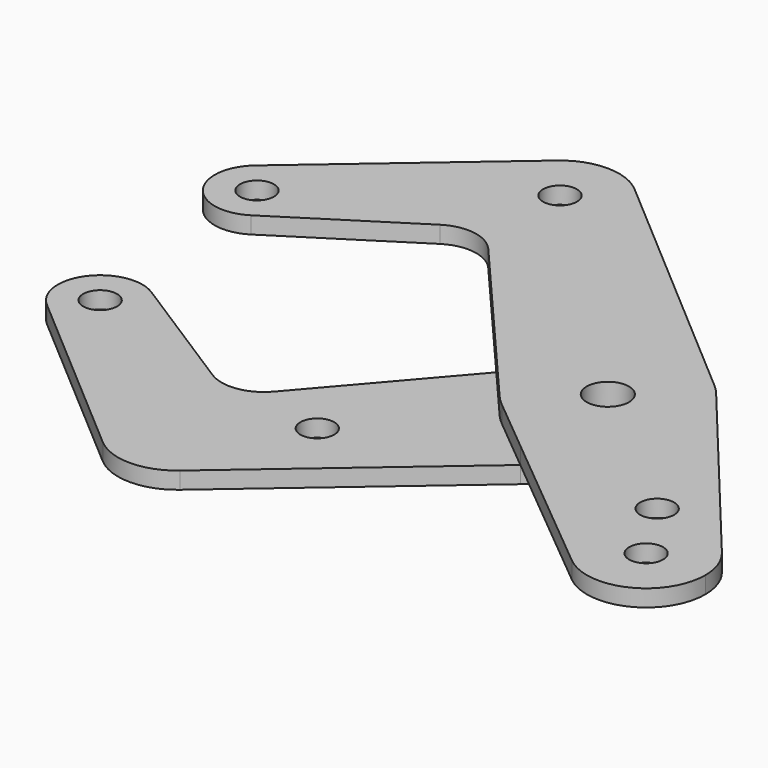
from build123d import *

# Parameters (mm, degrees)
F0_R     = 3.175
F0_R_2   = 3.9751
F1_DEPTH = 3.175
F2_DEPTH = 3.175


# Not quite as in the source:
# - after a boolean that leaves OpenCascade's solid faulty, fix() repairs it


with BuildPart() as f1:
    # F0 (on Top) → F1 (new body)
    with BuildSketch(Plane.XY):
        with BuildLine():
            Line((0.1954344954, -20.7710836138), (-10.1235074968, -12.2282550252))
            ThreePointArc((-10.1235074968, -12.2282550252), (-11.1192092809, -11.3304373246), (-12.0356034274, -10.3518054047))
            Line((-12.0356034274, -10.3518054047), (-20.9391765456, 0))
            Line((-20.9391765456, 0), (-42.5571087943, -25.134249466))
            ThreePointArc((-42.5571087943, -25.134249466), (-47.4235249822, -27.815033629), (-52.8569612369, -26.6546971654))
            Line((-52.8569612369, -26.6546971654), (-76.3196547531, -11.7034610596))
            ThreePointArc((-76.3196547531, -11.7034610596), (-73.6260110422, -14.5799404883), (-72.6477527528, -18.3973821792))
            ThreePointArc((-72.6477527528, -18.3973821792), (-77.2746501981, -25.611522251), (-85.7611554551, -24.4151838929))
            Line((-85.7611554551, -24.4151838929), (-52.1475443887, -53.3262030046))
            ThreePointArc((-52.1475443887, -53.3262030046), (-49.5361241819, -34.8014845049), (-33.7887806053, -44.9012806053))
            ThreePointArc((-33.7887806053, -44.9012806053), (-34.8014845049, -49.5361241819), (-37.655016822, -53.3262030046))
            Line((-37.655016822, -53.3262030046), (0.1954344954, -20.7710836138))
        make_face()
        with Locations((-30.2993841525, -30.2993841525)):
            Circle(F0_R, mode=Mode.SUBTRACT)
        with BuildLine():
            ThreePointArc((-52.1475443887, -53.3262030046), (-44.9012806053, -56.0137806053), (-37.655016822, -53.3262030046))
            ThreePointArc((-37.655016822, -53.3262030046), (-34.8014845049, -49.5361241819), (-33.7887806053, -44.9012806053))
            ThreePointArc((-33.7887806053, -44.9012806053), (-49.5361241819, -34.8014845049), (-52.1475443887, -53.3262030046))
        make_face()
        with BuildLine():
            ThreePointArc((-76.3196547531, -11.7034610596), (-86.9573903855, -13.664542837), (-85.7611554551, -24.4151838929))
            ThreePointArc((-85.7611554551, -24.4151838929), (-77.2746501981, -25.611522251), (-72.6477527528, -18.3973821792))
            ThreePointArc((-72.6477527528, -18.3973821792), (-73.6260110422, -14.5799404883), (-76.3196547531, -11.7034610596))
        make_face()
        with Locations((-80.5852527528, -18.3973821792)):
            Circle(F0_R, mode=Mode.SUBTRACT)
        with BuildLine():
            Line((0.1954344954, -20.7710836138), (10.3518055249, -12.0356033241))
            ThreePointArc((10.3518055249, -12.0356033241), (0.1493608613, -15.8742973493), (-10.1235074968, -12.2282550252))
            Line((-10.1235074968, -12.2282550252), (0.1954344954, -20.7710836138))
        make_face()
        with BuildLine():
            ThreePointArc((-12.0356034274, -10.3518054047), (-15.875, 6.76e-08), (-12.0356033393, 10.3518055072))
            Line((-12.0356033393, 10.3518055072), (-20.9391765456, 0))
            Line((-20.9391765456, 0), (-12.0356034274, -10.3518054047))
        make_face()
        with BuildLine():
            ThreePointArc((10.3518055249, -12.0356033241), (14.4282801766, -6.6212050373), (15.875, 0))
            ThreePointArc((15.875, 0), (14.9355142785, 5.3801522504), (12.2282550252, 10.1235074968))
            ThreePointArc((12.2282550252, 10.1235074968), (11.3304373246, 11.1192092809), (10.3518054047, 12.0356034274))
            ThreePointArc((10.3518054047, 12.0356034274), (-1.1906249326, 15.8302886035), (-12.0356033393, 10.3518055072))
            ThreePointArc((-12.0356033393, 10.3518055072), (-15.875, 6.76e-08), (-12.0356034274, -10.3518054047))
            ThreePointArc((-12.0356034274, -10.3518054047), (-11.1192092809, -11.3304373246), (-10.1235074968, -12.2282550252))
            ThreePointArc((-10.1235074968, -12.2282550252), (0.1493608613, -15.8742973493), (10.3518055249, -12.0356033241))
        make_face()
        Circle(F0_R_2, mode=Mode.SUBTRACT)
    extrude(amount=-F1_DEPTH)

    # F0 (on Top) → F2 (join)
    with BuildSketch(Plane.XY):
        with BuildLine():
            ThreePointArc((-12.0356033393, 10.3518055072), (-1.1906249326, 15.8302886035), (10.3518054047, 12.0356034274))
            Line((10.3518054047, 12.0356034274), (-37.655016822, 53.3262030046))
            ThreePointArc((-37.655016822, 53.3262030046), (-34.8014845049, 49.5361241819), (-33.7887806053, 44.9012806053))
            ThreePointArc((-33.7887806053, 44.9012806053), (-49.5361241819, 34.8014845049), (-52.1475443887, 53.3262030046))
            Line((-52.1475443887, 53.3262030046), (-85.7611554551, 24.4151838929))
            ThreePointArc((-85.7611554551, 24.4151838929), (-77.2746501981, 25.611522251), (-72.6477527528, 18.3973821792))
            ThreePointArc((-72.6477527528, 18.3973821792), (-73.6260112444, 14.5799401196), (-76.3196554623, 11.7034606077))
            Line((-76.3196554623, 11.7034606077), (-52.8569612369, 26.6546971654))
            ThreePointArc((-52.8569612369, 26.6546971654), (-47.4235249822, 27.815033629), (-42.5571087943, 25.134249466))
            Line((-42.5571087943, 25.134249466), (-20.9391765456, 0))
            Line((-20.9391765456, 0), (-12.0356033393, 10.3518055072))
        make_face()
        with BuildLine():
            ThreePointArc((-72.6477527528, 18.3973821792), (-77.2746501981, 25.611522251), (-85.7611554551, 24.4151838929))
            ThreePointArc((-85.7611554551, 24.4151838929), (-86.9573906362, 13.6645431745), (-76.3196554623, 11.7034606077))
            ThreePointArc((-76.3196554623, 11.7034606077), (-73.6260112444, 14.5799401196), (-72.6477527528, 18.3973821792))
        make_face()
        with Locations((-80.5852527528, 18.3973821792)):
            Circle(F0_R, mode=Mode.SUBTRACT)
        with BuildLine():
            ThreePointArc((-33.7887806053, 44.9012806053), (-34.8014845049, 49.5361241819), (-37.655016822, 53.3262030046))
            ThreePointArc((-37.655016822, 53.3262030046), (-44.9012806053, 56.0137806053), (-52.1475443887, 53.3262030046))
            ThreePointArc((-52.1475443887, 53.3262030046), (-49.5361241819, 34.8014845049), (-33.7887806053, 44.9012806053))
        make_face()
        with Locations((-44.9012806053, 44.9012806053)):
            Circle(F0_R, mode=Mode.SUBTRACT)
        with BuildLine():
            ThreePointArc((10.3518055249, -12.0356033241), (14.4282801766, -6.6212050373), (15.875, 0))
            ThreePointArc((15.875, 0), (14.9355142785, 5.3801522504), (12.2282550252, 10.1235074968))
            ThreePointArc((12.2282550252, 10.1235074968), (11.3304373246, 11.1192092809), (10.3518054047, 12.0356034274))
            ThreePointArc((10.3518054047, 12.0356034274), (-1.1906249326, 15.8302886035), (-12.0356033393, 10.3518055072))
            ThreePointArc((-12.0356033393, 10.3518055072), (-15.875, 6.76e-08), (-12.0356034274, -10.3518054047))
            ThreePointArc((-12.0356034274, -10.3518054047), (-11.1192092809, -11.3304373246), (-10.1235074968, -12.2282550252))
            ThreePointArc((-10.1235074968, -12.2282550252), (0.1493608613, -15.8742973493), (10.3518055249, -12.0356033241))
        make_face()
        Circle(F0_R_2, mode=Mode.SUBTRACT)
        with BuildLine():
            ThreePointArc((-12.0356034274, -10.3518054047), (-15.875, 6.76e-08), (-12.0356033393, 10.3518055072))
            Line((-12.0356033393, 10.3518055072), (-20.9391765456, 0))
            Line((-20.9391765456, 0), (-12.0356034274, -10.3518054047))
        make_face()
        with BuildLine():
            Line((0.1954344954, -20.7710836138), (10.3518055249, -12.0356033241))
            ThreePointArc((10.3518055249, -12.0356033241), (0.1493608613, -15.8742973493), (-10.1235074968, -12.2282550252))
            Line((-10.1235074968, -12.2282550252), (0.1954344954, -20.7710836138))
        make_face()
        with BuildLine():
            ThreePointArc((12.2282550252, 10.1235074968), (14.9355142785, 5.3801522504), (15.875, 0))
            ThreePointArc((15.875, 0), (14.4282801766, -6.6212050373), (10.3518055249, -12.0356033241))
            Line((10.3518055249, -12.0356033241), (0.1954344954, -20.7710836138))
            Line((0.1954344954, -20.7710836138), (28.8345692365, -44.4808030019))
            ThreePointArc((28.8345692365, -44.4808030019), (24.8320655021, -35.1980826181), (30.0059355892, -26.5136135964))
            ThreePointArc((30.0059355892, -26.5136135964), (37.6803722933, -24.9486796329), (44.4808030542, -28.8345692997))
            Line((44.4808030542, -28.8345692997), (12.2282550252, 10.1235074968))
        make_face()
        with BuildLine():
            ThreePointArc((31.490910058, -23.8257819975), (31.094979692, -25.361163699), (30.0059355892, -26.5136135964))
            ThreePointArc((30.0059355892, -26.5136135964), (25.536840424, -22.290400296), (31.490910058, -23.8257819975))
        make_face(mode=Mode.SUBTRACT)
        with BuildLine():
            ThreePointArc((47.0335244843, -35.9210244843), (46.3758844931, -32.1549179476), (44.4808030542, -28.8345692997))
            ThreePointArc((44.4808030542, -28.8345692997), (37.6803722933, -24.9486796329), (30.0059355892, -26.5136135964))
            ThreePointArc((30.0059355892, -26.5136135964), (24.8320655021, -35.1980826181), (28.8345692365, -44.4808030019))
            ThreePointArc((28.8345692365, -44.4808030019), (40.650687385, -45.9767663811), (47.0335244843, -35.9210244843))
        make_face()
        with Locations((35.9210244843, -35.9210244843)):
            Circle(F0_R, mode=Mode.SUBTRACT)
    extrude(amount=F2_DEPTH)

    add(f1.part.fix(), mode=Mode.REPLACE)


solid = f1.part
